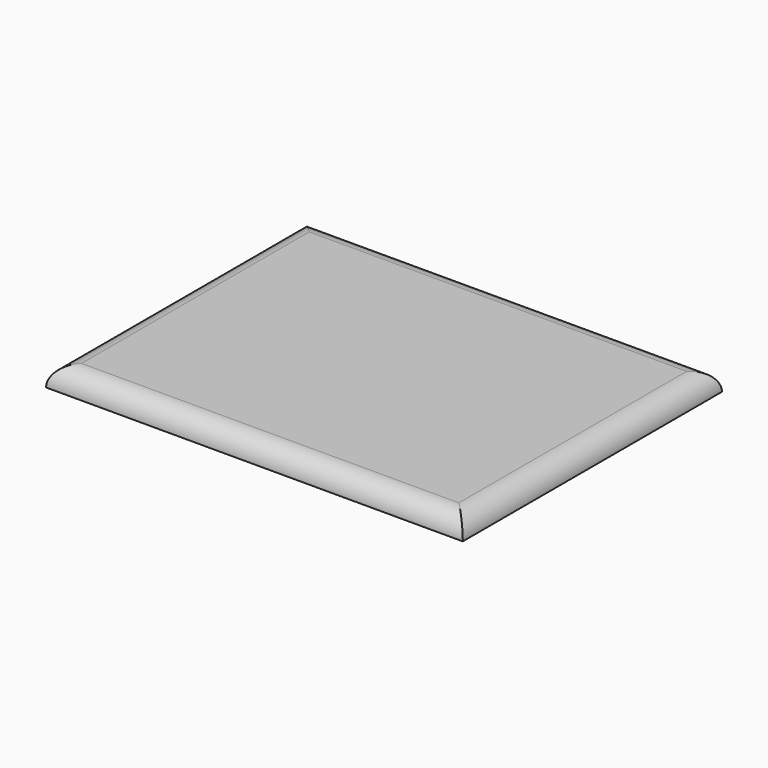
from build123d import *

# Parameters (mm, degrees)
F0_W     = 107.95
F0_H     = 83.9216
F1_DEPTH = 5.08
F2_R     = 5.07999


# Not quite as in the source:
# - a fillet or chamfer is up to 0.001 mm smaller than in the source, because OpenCascade refuses the exact size


with BuildPart() as f1:
    # F0 (on Top) → F1 (new body)
    with BuildSketch(Plane.XY):
        with Locations((1.8435493112, 6.7172771326)):
            Rectangle(F0_W, F0_H)
    extrude(amount=F1_DEPTH)

    # F2 (radius 5.08 in the source; OpenCascade refuses exactly that, so slightly less here)
    f2_edges = [f1.edges().sort_by_distance(p)[0] for p in [
        (1.843549, -35.243523, 5.08),
        (55.818549, 6.717277, 5.08),
        (-52.131451, 6.717277, 5.08),
        (1.843549, 48.678077, 5.08),
    ]]
    fillet(f2_edges, radius=F2_R)


solid = f1.part
